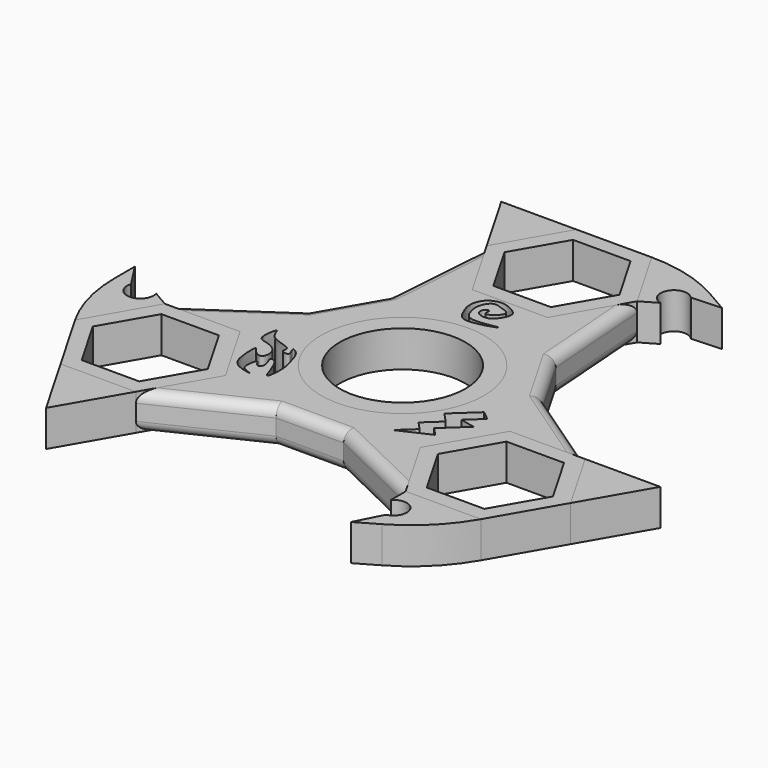
from build123d import *

# Parameters (mm, degrees)
F1_R     = 14.2875
F2_DEPTH = 6.35
F0_R     = 14.2875
F0_R_2   = 11.0236
F4_DEPTH = 6.35
F5_R     = 1.778


with BuildPart() as f2:
    # F1 (on Top) → F2 (new body)
    with BuildSketch(Plane.XY):
        with BuildLine():
            Line((-20.5516560741, 5.0371375), (-36.8377184556, -6.0452))
            Line((-36.8377184556, -6.0452), (-30.2459372272, -6.0452))
            ThreePointArc((-30.2459372272, -6.0452), (-22.1726869743, -9.3892497472), (-18.8286372272, -17.4625))
            ThreePointArc((-18.8286372272, -17.4625), (-19.217672238, -20.417514487), (-20.358265181, -23.1711496474))
            Line((-20.358265181, -23.1711496474), (-23.6541559988, -28.8798))
            Line((-23.6541559988, -28.8798), (-5.9135389997, -20.316825))
            Line((-5.9135389997, -20.316825), (5.9135389997, -20.316825))
            Line((5.9135389997, -20.316825), (23.6541559988, -28.8798))
            Line((23.6541559988, -28.8798), (20.3582654511, -23.1711501152))
            Line((20.3582654511, -23.1711501152), (17.0623747703, -17.4625))
            Line((17.0623747703, -17.4625), (20.3582651349, -11.7538504325))
            Line((20.3582651349, -11.7538504325), (23.6541559988, -6.0452))
            Line((23.6541559988, -6.0452), (30.2459372272, -6.0452))
            Line((30.2459372272, -6.0452), (36.8377184556, -6.0452))
            Line((36.8377184556, -6.0452), (20.5516560741, 5.0371375))
            Line((20.5516560741, 5.0371375), (14.6381170744, 15.2796875))
            Line((14.6381170744, 15.2796875), (13.1835624568, 34.925))
            Line((13.1835624568, 34.925), (9.8876717015, 29.2163497555))
            Line((9.8876717015, 29.2163497555), (6.5917812284, 23.5077))
            Line((6.5917812284, 23.5077), (0, 23.5077))
            Line((0, 23.5077), (-6.5917812284, 23.5077))
            Line((-6.5917812284, 23.5077), (-9.8876721491, 29.2163505308))
            Line((-9.8876721491, 29.2163505308), (-13.1835624568, 34.925))
            Line((-13.1835624568, 34.925), (-14.6381170744, 15.2796875))
            Line((-14.6381170744, 15.2796875), (-20.5516560741, 5.0371375))
        make_face()
        Circle(F1_R, mode=Mode.SUBTRACT)
    extrude(amount=F2_DEPTH)

    # F3 (on Top) → F4 (cut)
    with BuildSketch(Plane.XY):
        Polygon((18.9453903586, -8.1055236718), (16.3444373757, -7.5413030572), (18.9453903586, -5.1308954337), (17.3724049037, -3.8256528787), (13.3630285141, -7.5413030572), (14.9820335209, -9.2882921808), (12.2534246479, -11.8170036465), (13.6017040761, -13.2718660383), (10.8589707764, -15.8136671774), (16.3444373757, -13.2718660383), (14.9820335209, -11.8170036465), align=None)
        with BuildLine():
            add(Edge.make_bspline(
                [(-0.8817947237, 20.0824197382), (-1.0075664363, 20.2238511955), (-1.8282999289, 19.8987410627), (-1.8510807176, 18.4204917331), (0.1154141916, 17.9731951571), (1.3992341464, 18.6686879762), (2.7805172326, 21.2638739316), (1.1775048058, 22.3395891298), (-0.7563332235, 23.2779789446), (-3.4780762373, 22.4050316842), (-4.3115834076, 19.6753132276), (-3.4286001584, 17.5514412276), (-2.2345013378, 14.8906729818), (6.4713090932, 18.0054024378), (-1.922048173, 15.7706909758), (-2.7430823494, 18.4412394848), (-3.1678669838, 20.1899616032), (-1.8896002645, 22.5060398746), (-0.095997299, 21.7314951338), (2.1515170738, 21.0754922038), (0.1405906438, 19.0401476636), (-1.0339454481, 18.9710523168), (-0.7453889895, 19.9290302249), (-0.8817947237, 20.0824197382)],
                knots=[0, 0, 0, 0, 0.0292242291, 0.0652724413, 0.108923933, 0.1500467643, 0.2031690575, 0.2452221963, 0.2945595542, 0.3482072254, 0.4018548917, 0.4527970409, 0.5060024489, 0.5818087159, 0.6540115837, 0.705234834, 0.7511548795, 0.7999852729, 0.8450494925, 0.888386887, 0.9381558104, 0.9683048569, 1, 1, 1, 1], degree=3))
        make_face()
        with BuildLine():
            add(Edge.make_bspline(
                [(-14.9852787245, -14.803975754), (-14.962304639, -14.7710058159), (-16.0751064868, -14.4487676827), (-16.9493376323, -13.7844407153), (-16.4153619195, -10.5756747049), (-15.5799569425, -12.9279508378), (-14.3806627568, -11.6176411833), (-15.8241772837, -9.5012222196), (-14.4294463891, -9.7145071424), (-13.6142068864, -11.4573431251), (-13.2482714067, -12.4512081263), (-12.4537024099, -14.9392992259), (-11.9819647052, -10.7861534353), (-12.7985167121, -8.3243550918), (-13.4313940545, -6.1812801335), (-15.2851630075, -5.1110667924), (-13.6159495138, -7.4338752765), (-15.9115240061, -7.1069026674), (-14.7998378074, -5.405651807), (-19.4457689348, -5.1471537646), (-19.8688721794, -1.742664042), (-20.4449161419, -4.2983598335), (-20.2522653632, -6.0932530851), (-18.6430682396, -6.2331643715), (-16.1556892371, -7.415318527), (-16.4603369048, -10.4034326443), (-18.2958958989, -9.5294161962), (-19.1406427169, -7.6608606548), (-19.0327624107, -11.9464988775), (-18.0715793146, -14.3266515145), (-15.0224819232, -14.8573657859), (-14.9852787245, -14.803975754)],
                knots=[0, 0, 0, 0, 0.0256101455, 0.0550542613, 0.0921947156, 0.1206410575, 0.1466940011, 0.1835440079, 0.2048757742, 0.2405975701, 0.2714432733, 0.3021944228, 0.3455278657, 0.3914057237, 0.4314078855, 0.4580219051, 0.4896714886, 0.5172375148, 0.543531976, 0.5943763459, 0.6312122696, 0.66389277, 0.6983545837, 0.7293098495, 0.7714457944, 0.8086318082, 0.8406120839, 0.8676550288, 0.9130852515, 0.9585280846, 1, 1, 1, 1], degree=3))
        make_face()
        Polygon((17.0623747703, -17.4625), (23.6541559988, -28.8798), (36.8377184556, -28.8798), (43.429499684, -17.4625), (36.8377184556, -6.0452), (23.6541559988, -6.0452), align=None)
    extrude(amount=F4_DEPTH, mode=Mode.SUBTRACT)

    # F5
    f5_edges = [f2.edges().sort_by_distance(p)[0] for p in [
        (13.91084, 25.102344, 6.35),
        (17.594887, 10.158412, 6.35),
        (28.694687, -0.504031, 6.35),
        (13.91084, 25.102344, 0),
        (17.594887, 10.158412, 0),
        (28.694687, -0.504031, 0),
        (-13.91084, 25.102344, 6.35),
        (-17.594887, 10.158413, 6.35),
        (-28.694687, -0.504031, 6.35),
        (-17.594887, 10.158413, 0),
        (-13.91084, 25.102344, 0),
        (-28.694687, -0.504031, 0),
        (0, -20.316825, 0),
        (-14.783847, -24.598312, 6.35),
        (-14.783847, -24.598312, 0),
        (0, -20.316825, 6.35),
        (14.783847, -24.598312, 6.35),
        (14.783847, -24.598312, 0),
    ]]
    fillet(f5_edges, radius=F5_R)


with BuildPart() as f2b:
    # F1 (on Top) → F2, piece 2 (new body)
    with BuildSketch(Plane.XY):
        Polygon((-19.7753436853, 46.3423), (-13.1835624568, 34.925), (-9.8876720638, 40.6336496169), (-6.5917812284, 46.3423), align=None)
    extrude(amount=F2_DEPTH)


with BuildPart() as f2c:
    # F1 (on Top) → F2, piece 3 (new body)
    with BuildSketch(Plane.XY):
        with BuildLine():
            ThreePointArc((19.7168434682, 42.8056682621), (13.3883800625, 45.4426505756), (6.5917812284, 46.3423))
            Line((6.5917812284, 46.3423), (9.8876717761, 40.6336501152))
            Line((9.8876717761, 40.6336501152), (13.1835624568, 34.925))
            Line((13.1835624568, 34.925), (15.9968403488, 36.5492467482))
            ThreePointArc((15.9968403488, 36.5492467482), (14.4966445581, 39.9883584633), (18.2287384143, 40.3750783203))
            Line((18.2287384143, 40.3750783203), (23.4646089375, 40.6418948595))
            Line((23.4646089375, 40.6418948595), (19.7168434682, 42.8056682621))
        make_face()
    extrude(amount=F2_DEPTH)


with BuildPart() as f2d:
    # F1 (on Top) → F2, piece 4 (new body)
    with BuildSketch(Plane.XY):
        Polygon((40.1336093195, -11.7538504325), (43.429499684, -17.4625), (50.0212809124, -6.0452), (36.8377184556, -6.0452), align=None)
    extrude(amount=F2_DEPTH)


with BuildPart() as f2e:
    # F1 (on Top) → F2, piece 5 (new body)
    with BuildSketch(Plane.XY):
        with BuildLine():
            Line((30.2459372272, -28.8798), (23.6541559988, -28.8798))
            Line((23.6541559988, -28.8798), (23.6541559988, -32.1282934964))
            ThreePointArc((23.6541559988, -32.1282934964), (27.3826120058, -32.5486416886), (25.851474298, -35.9740897059))
            Line((25.851474298, -35.9740897059), (23.4646089375, -40.6418948595))
            Line((23.4646089375, -40.6418948595), (27.2123744068, -38.4781214569))
            ThreePointArc((27.2123744068, -38.4781214569), (32.6602997825, -34.3160025375), (36.8377184556, -28.8798))
            Line((36.8377184556, -28.8798), (30.2459372272, -28.8798))
        make_face()
    extrude(amount=F2_DEPTH)


with BuildPart() as f2f:
    # F1 (on Top) → F2, piece 6 (new body)
    with BuildSketch(Plane.XY):
        Polygon((-23.6541559988, -28.8798), (-30.2459372272, -28.8798), (-36.8377184556, -28.8798), (-30.2459372272, -40.2971), align=None)
    extrude(amount=F2_DEPTH)


with BuildPart() as f2g:
    # F1 (on Top) → F2, piece 7 (new body)
    with BuildSketch(Plane.XY):
        with BuildLine():
            Line((-40.1336093656, -11.7538505124), (-36.8377184556, -6.0452))
            Line((-36.8377184556, -6.0452), (-39.6509963475, -4.4209532518))
            ThreePointArc((-39.6509963475, -4.4209532518), (-41.8792565639, -7.4397167747), (-44.0802127123, -4.4009886144))
            Line((-44.0802127123, -4.4009886144), (-46.929217875, 0))
            Line((-46.929217875, 0), (-46.929217875, -4.3275468051))
            ThreePointArc((-46.929217875, -4.3275468051), (-46.048679845, -11.1266480381), (-43.429499684, -17.4625))
            Line((-43.429499684, -17.4625), (-40.1336093656, -11.7538505124))
        make_face()
    extrude(amount=F2_DEPTH)


with BuildPart() as f2h:
    # F0 (on Top) → F2, piece 8 (new body)
    with BuildSketch(Plane.XY):
        Polygon((-6.5917812284, 23.5077), (6.5917812284, 23.5077), (13.1835624568, 34.925), (6.5917812284, 46.3423), (-6.5917812284, 46.3423), (-13.1835624568, 34.925), align=None)
        Polygon((10.0819790757, 34.925), (5.0409895379, 26.19375), (-5.0409895379, 26.19375), (-10.0819790757, 34.925), (-5.0409895379, 43.65625), (5.0409895379, 43.65625), align=None, mode=Mode.SUBTRACT)
    extrude(amount=F2_DEPTH)


with BuildPart() as f2i:
    # F0 (on Top) → F2, piece 9 (new body)
    with BuildSketch(Plane.XY):
        Polygon((43.429499684, -17.4625), (36.8377184556, -6.0452), (23.6541559988, -6.0452), (17.0623747703, -17.4625), (23.6541559988, -28.8798), (36.8377184556, -28.8798), align=None)
        Polygon((35.286926765, -26.19375), (25.2049476893, -26.19375), (20.1639581514, -17.4625), (25.2049476893, -8.73125), (35.286926765, -8.73125), (40.3279163029, -17.4625), align=None, mode=Mode.SUBTRACT)
    extrude(amount=F2_DEPTH)


with BuildPart() as f2j:
    # F0 (on Top) → F2, piece 10 (new body)
    with BuildSketch(Plane.XY):
        Polygon((-36.8377184556, -28.8798), (-23.6541559988, -28.8798), (-17.0623747703, -17.4625), (-23.6541559988, -6.0452), (-36.8377184556, -6.0452), (-43.429499684, -17.4625), align=None)
        Polygon((-40.3279163029, -17.4625), (-35.286926765, -8.73125), (-25.2049476893, -8.73125), (-20.1639581514, -17.4625), (-25.2049476893, -26.19375), (-35.286926765, -26.19375), align=None, mode=Mode.SUBTRACT)
    extrude(amount=F2_DEPTH)


with BuildPart() as f2k:
    # F0 (on Top) → F2, piece 11 (new body)
    with BuildSketch(Plane.XY):
        Circle(F0_R)
        Circle(F0_R_2, mode=Mode.SUBTRACT)
    extrude(amount=F2_DEPTH)


solid = Compound([f2.part, f2b.part, f2c.part, f2d.part, f2e.part, f2f.part, f2g.part, f2h.part, f2i.part, f2j.part, f2k.part])
